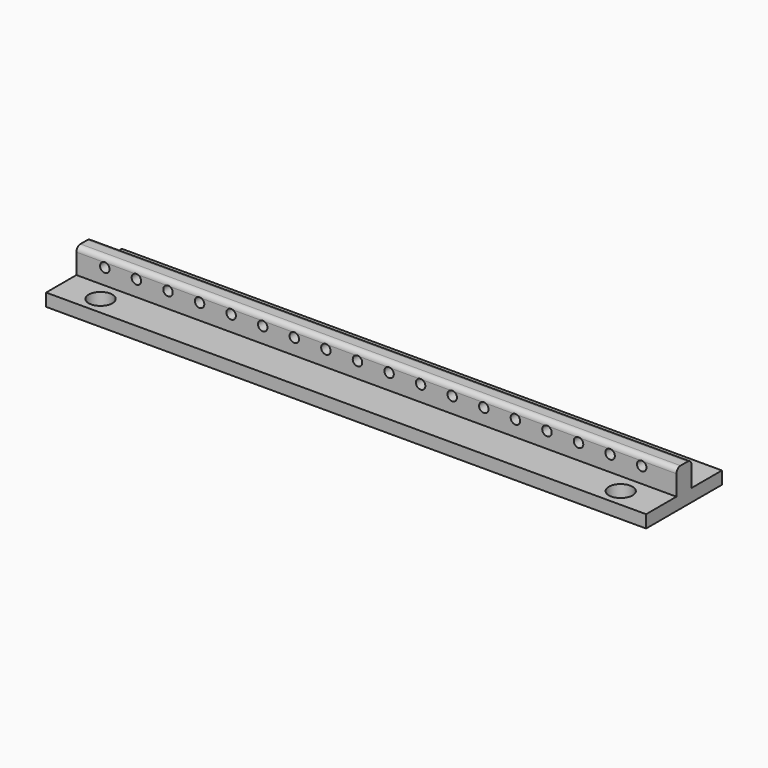
from build123d import *

# Parameters (mm, degrees)
F0_W        = 241.3
F0_H        = 38.1
F1_DEPTH    = 5.08
F2_W        = 241.3
F2_H        = 7.62
F3_DEPTH    = 10.16
F4_R        = 1.905
F5_DEPTH    = 22.861
F6_R        = 4.7625
F7_R        = 4.7625
F8_DEPTH    = 5.081
F9_T1_DEPTH = 251.46


# Not quite as in the source:
# - a fillet or chamfer that OpenCascade refuses, or shapes differently, is made with other operations: its cross-section is extruded or revolved along the edge and cut away or added


with BuildPart() as f1:
    # F0 (on Top) → F1 (new body)
    with BuildSketch(Plane.XY):
        with Locations((-10.1314700298, 19.05)):
            Rectangle(F0_W, F0_H)
    extrude(amount=F1_DEPTH)

    # F2 (on face) → F3 (join)
    with BuildSketch(Plane.XY.offset(5.08)):
        with Locations((-10.1314700298, 19.05)):
            Rectangle(F2_W, F2_H)
    extrude(amount=F3_DEPTH)

    # F4 (on face) → F5 (cut, through all)
    with BuildSketch(Plane.XZ.offset(-15.24)):
        with Locations((-119.3514700298, 11.43)):
            Circle(F4_R)
        with Locations((-106.6514700298, 11.43)):
            Circle(F4_R)
        with Locations((-93.9514700298, 11.43)):
            Circle(F4_R)
        with Locations((-81.2514700298, 11.43)):
            Circle(F4_R)
        with Locations((-68.5514700298, 11.43)):
            Circle(F4_R)
        with Locations((-55.8514700298, 11.43)):
            Circle(F4_R)
        with Locations((-43.1514700298, 11.43)):
            Circle(F4_R)
        with Locations((-30.4514700298, 11.43)):
            Circle(F4_R)
        with Locations((-17.7514700298, 11.43)):
            Circle(F4_R)
        with Locations((-5.0514700298, 11.43)):
            Circle(F4_R)
        with Locations((7.6485299702, 11.43)):
            Circle(F4_R)
        with Locations((20.3485299702, 11.43)):
            Circle(F4_R)
        with Locations((33.0485299702, 11.43)):
            Circle(F4_R)
        with Locations((45.7485299702, 11.43)):
            Circle(F4_R)
        with Locations((58.4485299702, 11.43)):
            Circle(F4_R)
        with Locations((71.1485299702, 11.43)):
            Circle(F4_R)
        with Locations((83.8485299702, 11.43)):
            Circle(F4_R)
        with Locations((96.5485299702, 11.43)):
            Circle(F4_R)
    extrude(amount=-F5_DEPTH, mode=Mode.SUBTRACT)

    # F6 (on face) + F7 (on face) → F8 (cut, through all)
    with BuildSketch(Plane.XY.offset(5.08)):
        with Locations((-114.719107688, 30.7975)):
            Circle(F6_R)
        with Locations((94.4530299702, 30.7975)):
            Circle(F6_R)
    with BuildSketch(Plane.XY.offset(5.08)):
        with Locations((-114.719107688, 7.3025)):
            Circle(F7_R)
        with Locations((94.4561676284, 7.3025)):
            Circle(F7_R)
    extrude(amount=-F8_DEPTH, mode=Mode.SUBTRACT)

    # F9: fillet of radius 2.032 on 2 edges, made by hand

    # F9_s2 → F9_t1 (cut)
    with BuildSketch(Plane.YZ.offset(-135.8614700298)):
        with BuildLine():
            ThreePointArc((15.24, 13.208), (15.8351590206, 14.6448409794), (17.272, 15.24))
            Line((17.272, 15.24), (15.24, 15.24))
            Line((15.24, 15.24), (15.24, 13.208))
        make_face()
        with BuildLine():
            ThreePointArc((20.828, 15.24), (22.2648409794, 14.6448409794), (22.86, 13.208))
            Line((22.86, 13.208), (22.86, 15.24))
            Line((22.86, 15.24), (20.828, 15.24))
        make_face()
    extrude(amount=F9_T1_DEPTH, mode=Mode.SUBTRACT)


solid = f1.part
